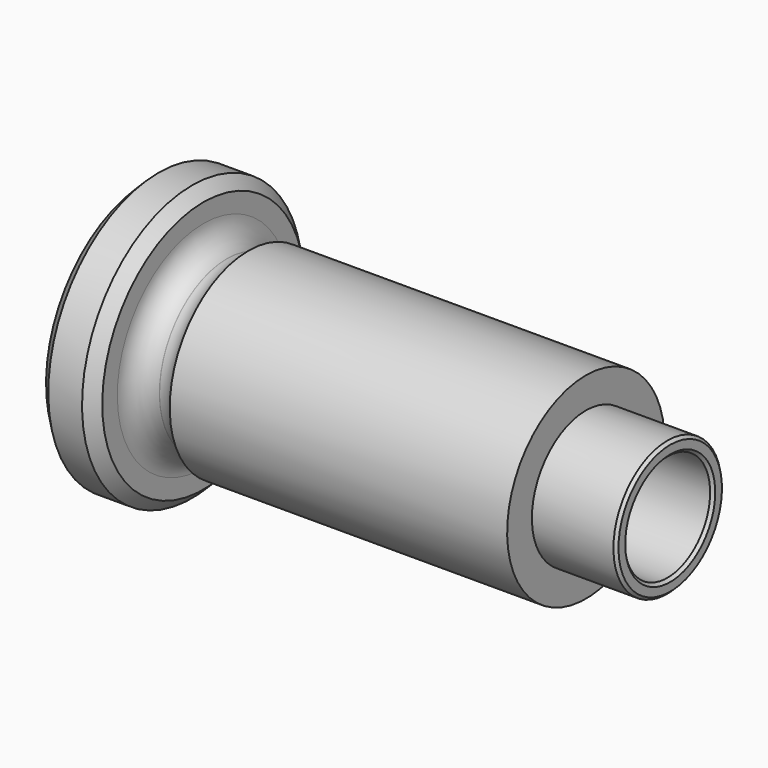
from build123d import *

# Parameters (mm, degrees)
F3_SIZE = 2
F4_SIZE = 0.5


# Not quite as in the source:
# - a fillet or chamfer that OpenCascade refuses, or shapes differently, is made with other operations: its cross-section is extruded or revolved along the edge and cut away or added


with BuildPart() as f1:
    # F0 (on Front) → F1 (revolve)
    with BuildSketch(Plane.XZ):
        Polygon((0, 24.5), (0, 0), (19, 0), (19, 9.5), (93, 9.5), (93, 12), (78, 12), (78, 17.5), (18, 17.5), (18, 15), (10, 15), (10, 24.5), align=None)
    revolve(axis=Axis((9.5, 0, 0), (-1, 0, 0)))

    # F2: fillet of radius 4.15 on 2 edges, made by hand

    # F2_s1 → F2_t2 (revolve)
    with BuildSketch(Plane.XZ):
        with BuildLine():
            ThreePointArc((14.15, 15), (11.2155068581, 16.2155068581), (10, 19.15))
            Line((10, 19.15), (10, 15))
            Line((10, 15), (14.15, 15))
        make_face()
    revolve(axis=Axis((10, 0, 0), (-1, 0, 0)))

    # F2_s3 → F2_t4 (revolve)
    with BuildSketch(Plane.XZ):
        with BuildLine():
            ThreePointArc((18, 17.5), (16.4697218419, 15.6808502483), (14.1921134471, 15))
            Line((14.1921134471, 15), (18, 15))
            Line((18, 15), (18, 17.5))
        make_face()
    revolve(axis=Axis((18, 0, 0), (-1, 0, 0)))

    # F3
    f3_edges = [f1.edges().sort_by_distance(p)[0] for p in [
        (0, 0, -24.5),
        (10, 0, -24.5),
    ]]
    chamfer(f3_edges, length=F3_SIZE)

    # F4
    f4_edges = [f1.edges().sort_by_distance(p)[0] for p in [
        (93, 0, -12),
        (93, 0, -9.5),
    ]]
    chamfer(f4_edges, length=F4_SIZE)


solid = f1.part
